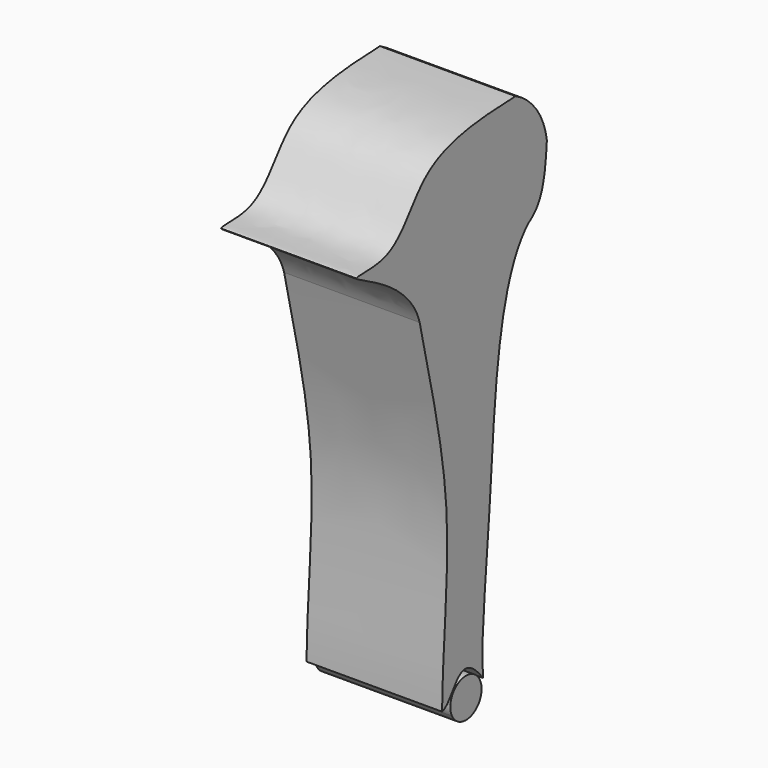
from build123d import *

# Parameters (mm, degrees)
F1_DEPTH = 50.8


with BuildPart() as f1:
    # F0 (on Right) → F1 (new body)
    with BuildSketch(Plane.YZ):
        with BuildLine():
            add(Edge.make_bspline(
                [(-29.6350651787, 80.786230328), (4.2160376009, 69.9020710126), (38.0671403805, 59.0179116973), (50.9450534633, 66.4803572774)],
                knots=[0, 0, 0, 0, 0.6430590338, 0.6430590338, 0.6430590338, 0.6430590338], degree=3))
            ThreePointArc((50.9450534633, 66.4803572774), (54.6649643889, 70.68743111), (57.4397514742, 75.5698243918))
            add(Edge.make_bspline(
                [(57.4397514742, 75.5698243918), (58.7432663916, 79.9010257326), (59.1044894484, 85.0565106809), (59.4657125052, 90.2119956291)],
                knots=[0.8121232615, 0.8121232615, 0.8121232615, 0.8121232615, 1, 1, 1, 1], degree=3))
            ThreePointArc((59.4657125052, 90.2119956291), (54.6535895657, 102.2714788741), (44.7917432786, 110.7172855929))
            add(Edge.make_bspline(
                [(44.7917432786, 110.7172855929), (26.8489347918, 110.0752117141), (0.5734328089, 108.1092295228), (-10.2101926789, 78.7917675971), (-29.8744603488, 81.768573432), (-29.6350651787, 80.786230328)],
                knots=[0, 0, 0, 0, 0.3004250191, 0.5376572536, 0.7103136826, 0.7103136826, 0.7103136826, 0.7103136826], degree=3))
        make_face()
        with BuildLine():
            add(Edge.make_bspline(
                [(50.9450534633, 66.4803572774), (36.3766547955, 53.0931885378), (34.1317834651, -18.0947327184), (28.3926753236, -62.5393411205), (29.5680372394, -75.0765348892)],
                knots=[0, 0, 0, 0, 0.5471772578, 1, 1, 1, 1], degree=3))
            add(Edge.make_bspline(
                [(-29.6350651787, 80.786230328), (4.2160376009, 69.9020710126), (38.0671403805, 59.0179116973), (50.9450534633, 66.4803572774)],
                knots=[0, 0, 0, 0, 0.6430590338, 0.6430590338, 0.6430590338, 0.6430590338], degree=3))
            add(Edge.make_bspline(
                [(-29.6350651787, 80.786230328), (-29.2334033024, 79.1380359465), (-4.8401590719, 71.1946062517), (-0.1259154906, 54.301901374)],
                knots=[0.7103136826, 0.7103136826, 0.7103136826, 0.7103136826, 1, 1, 1, 1], degree=3))
            add(Edge.make_bspline(
                [(-0.1259154906, 54.301901374), (5.1043563051, 31.124734176), (16.9751424435, -12.4998767043), (10.5838589864, -56.8508905259), (10.3848146308, -78.3914512205)],
                knots=[0, 0, 0, 0, 0.5066770175, 1, 1, 1, 1], degree=3))
            add(Edge.make_bspline(
                [(10.3848146308, -78.3914512205), (16.348344002, -76.7541756137), (17.8574419675, -59.6243200311), (29.5680372394, -75.0765348892)],
                knots=[0, 0, 0, 0, 19.4675293742, 19.4675293742, 19.4675293742, 19.4675293742], degree=3))
        make_face()
        with BuildLine():
            ThreePointArc((57.4397514742, 75.5698243918), (54.6649643889, 70.68743111), (50.9450534633, 66.4803572774))
            add(Edge.make_bspline(
                [(50.9450534633, 66.4803572774), (54.3307370698, 68.4422807275), (56.2667603712, 71.6723157636), (57.4397514742, 75.5698243918)],
                knots=[0.6430590338, 0.6430590338, 0.6430590338, 0.6430590338, 0.8121232615, 0.8121232615, 0.8121232615, 0.8121232615], degree=3))
        make_face()
    extrude(amount=F1_DEPTH)


with BuildPart() as f1b:
    # F0 (on Right) → F1, piece 2 (new body)
    with BuildSketch(Plane.YZ):
        with BuildLine():
            Line((14.2522070165, -77.7231546345), (28.1996788547, -75.3129911744))
            ThreePointArc((28.1996788547, -75.3129911744), (20.3018620607, -71.1704721329), (14.2522070165, -77.7231546345))
        make_face()
        with BuildLine():
            ThreePointArc((28.8776664165, -78.3914512205), (28.706162596, -76.8153338875), (28.1996788547, -75.3129911744))
            Line((28.1996788547, -75.3129911744), (14.2522070165, -77.7231546345))
            ThreePointArc((14.2522070165, -77.7231546345), (14.3442995311, -79.7264502405), (14.9760174426, -81.6297649273))
            ThreePointArc((14.9760174426, -81.6297649273), (22.3719895847, -85.673164369), (28.6799543824, -80.0821838572))
            ThreePointArc((28.6799543824, -80.0821838572), (28.8280705758, -79.2425779586), (28.8776664165, -78.3914512205))
        make_face()
    extrude(amount=F1_DEPTH)


solid = Compound([f1.part, f1b.part])
